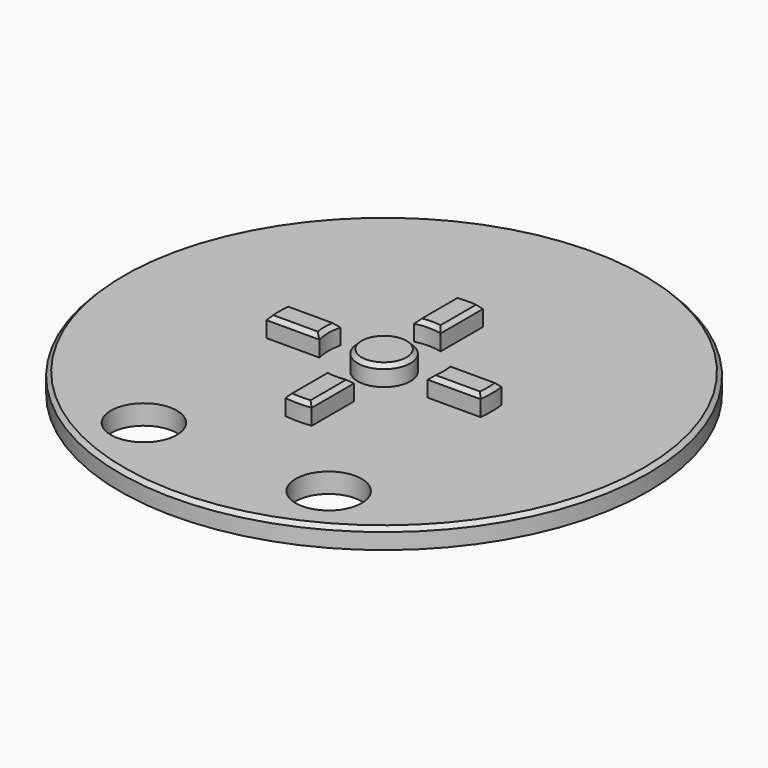
from build123d import *

# Parameters (mm, degrees)
F0_R     = 20
F1_DEPTH = 1.5
F2_D     = 5
F2_DEPTH = 20.381
F2_TIP   = 1.5021515476
F3_R     = 2
F4_DEPTH = 3
F5_SIZE  = 0.3


# Not quite as in the source:
# - a pattern or mirror of a feature is missing from the dataset's text; its kind, count and spacing are read off the source's solid


with BuildPart() as f1:
    # F0 (on Top) → F1 (new body)
    with BuildSketch(Plane.XY):
        Circle(F0_R)
    extrude(amount=F1_DEPTH)

    # F2
    with Locations(Plane(origin=(0, 0, 0), x_dir=(1, 0, 0), z_dir=(0, 0, -1))):
        with Locations((-7, 14)):
            f2 = Hole(F2_D / 2, depth=F2_DEPTH)
            with Locations((0, 0, -(F2_DEPTH + F2_TIP / 2))):  # 118° drill point
                Cone(0, F2_D / 2, F2_TIP, mode=Mode.SUBTRACT)

    # F2_copies: F2 across plane
    add(f2.mirror(Plane(origin=(0, 0, 0), x_dir=(0, 0, 1), z_dir=(1, 0, 0))), mode=Mode.SUBTRACT)

    # F3 (on Top) → F4 (join)
    with BuildSketch(Plane.XY):
        with BuildLine():
            Line((-4.104842454, 1.0004466142), (-8.104842454, 1.0004466142))
            ThreePointArc((-8.104842454, 1.0004466142), (-8.1663556518, 0), (-8.104842454, -1.0004466142))
            Line((-8.104842454, -1.0004466142), (-4.104842454, -1.0004466142))
            ThreePointArc((-4.104842454, -1.0004466142), (-4.225, 0), (-4.104842454, 1.0004466142))
        make_face()
        with BuildLine():
            ThreePointArc((1, 8.1048975707), (0, 8.1663556518), (-1, 8.1048975707))
            Line((-1, 8.1048975707), (-1, 4.1049512786))
            ThreePointArc((-1, 4.1049512786), (0, 4.225), (1, 4.1049512786))
            Line((1, 4.1049512786), (1, 8.1048975707))
        make_face()
        with BuildLine():
            Line((4.104842454, -1.0004466142), (8.104842454, -1.0004466142))
            ThreePointArc((8.104842454, -1.0004466142), (8.1663556518, 0), (8.104842454, 1.0004466142))
            Line((8.104842454, 1.0004466142), (4.104842454, 1.0004466142))
            ThreePointArc((4.104842454, 1.0004466142), (4.225, 0), (4.104842454, -1.0004466142))
        make_face()
        with BuildLine():
            ThreePointArc((-1, -8.1048975707), (0, -8.1663556518), (1, -8.1048975707))
            Line((1, -8.1048975707), (1, -4.1049512786))
            ThreePointArc((1, -4.1049512786), (0, -4.225), (-1, -4.1049512786))
            Line((-1, -4.1049512786), (-1, -8.1048975707))
        make_face()
        Circle(F3_R)
    extrude(amount=F4_DEPTH)

    # F5
    f5_edges = [f1.edges().sort_by_distance(p)[0] for p in [
        (-2, 0, 3),
        (0, 8.166356, 3),
        (-1, 6.104924, 3),
        (0, 4.225, 3),
        (1, 6.104924, 3),
        (6.104842, -1.000447, 3),
        (8.166356, 0, 3),
        (6.104842, 1.000447, 3),
        (4.225, 0, 3),
        (1, -6.104924, 3),
        (0, -4.225, 3),
        (-1, -6.104924, 3),
        (0, -8.166356, 3),
        (-6.104842, 1.000447, 3),
        (-8.166356, 0, 3),
        (-6.104842, -1.000447, 3),
        (-4.225, 0, 3),
        (-20, 0, 1.5),
    ]]
    chamfer(f5_edges, length=F5_SIZE)


solid = f1.part
